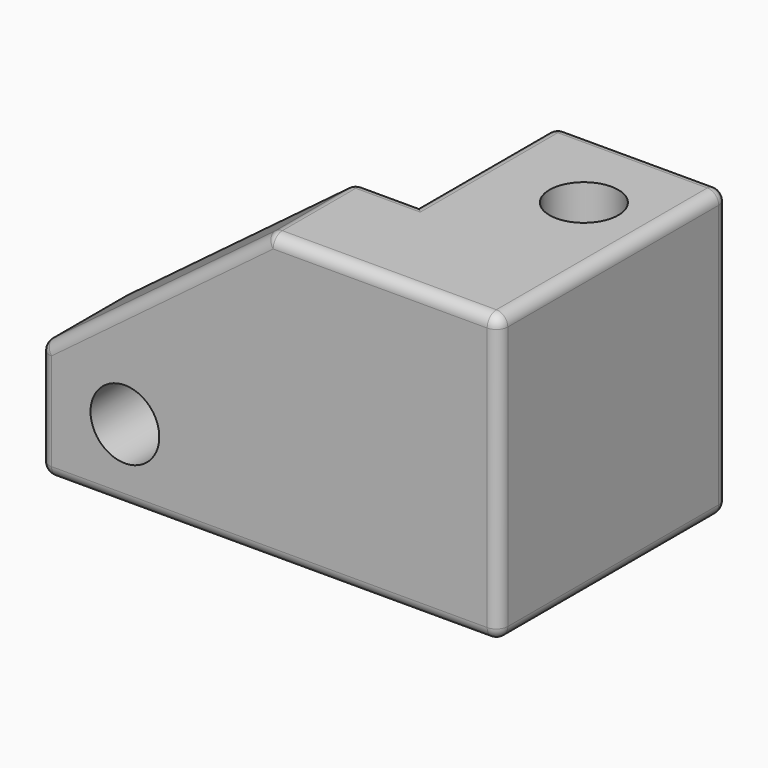
from build123d import *

# Parameters (mm, degrees)
F0_W          = 203.2
F0_H          = 127
F1_DEPTH      = 127
F3_DEPTH      = 76.2
F3_DEPTH_BACK = 76.2
F4_DEPTH      = 25.4
F5_SIZE2      = 101.6
F5_SIZE       = 76.2
F6_R          = 5.08
F7_R          = 15.24
F8_DEPTH      = 51.054
F9_R          = 15.24
F10_DEPTH     = 128.27


with BuildPart() as f1:
    # F0 (on Front) → F1 (new body)
    with BuildSketch(Plane.XZ):
        Rectangle(F0_W, F0_H)
    extrude(amount=F1_DEPTH)

    # F2 (on Front) → F3 (cut, two sides)
    with BuildSketch(Plane.XZ) as f3_sk:
        Polygon((25.2138410211, 63.1450035885), (-101.7861589789, 63.1450035885), (-101.7861589789, -63.8549964115), (-25.5861589789, -63.8549964115), (-25.5861589789, 12.3450035885), (25.2138410211, 12.3450035885), align=None)
    extrude(amount=-F3_DEPTH, mode=Mode.SUBTRACT)
    extrude(f3_sk.sketch, amount=F3_DEPTH_BACK, mode=Mode.SUBTRACT)

    # F4 (cut): a face of the model
    f4_faces = [f1.faces().sort_by_distance(p)[0] for p in [
        (-38.1930794895, -38.1, 63.1450035885),
    ]]
    extrude(f4_faces, amount=-F4_DEPTH, mode=Mode.SUBTRACT)

    # F5
    f5_edges = [f1.edges().sort_by_distance(p)[0] for p in [
        (-101.6, -101.6, 63.5),
    ]]
    f5_side = f1.faces().sort_by_distance((-101.6, -101.6, 0))[0]
    chamfer(f5_edges, length=F5_SIZE, length2=F5_SIZE2, reference=f5_side)

    # F6
    f6_edges = [f1.edges().sort_by_distance(p)[0] for p in [
        (25.213841, 0, 37.922502),
        (63.406921, 0, 63.5),
        (-0.186159, 0, 12.345004),
        (-25.586159, -38.1, 12.345004),
        (-101.6, -101.6, -12.7),
        (0, -101.6, 63.5),
        (101.6, 0, 0),
        (38.006921, 0, -63.5),
        (-25.586159, -38.1, -63.5),
        (-63.593079, -76.2, -63.5),
        (-101.6, -101.6, -63.5),
        (50.8, -127, 63.5),
        (-50.8, -127, 25.4),
        (101.6, -127, 0),
        (-101.6, -127, -38.1),
        (0, -127, -63.5),
        (-50.8, -76.2, 25.4),
        (101.6, -63.5, 63.5),
        (101.6, -63.5, -63.5),
        (12.606921, -76.2, 63.5),
        (25.213841, -38.1, 63.5),
    ]]
    fillet(f6_edges, radius=F6_R)

    # F7 (on face) → F8 (cut)
    with BuildSketch(Plane(origin=(0, -76.2, 0), x_dir=(-1, 0, 0), z_dir=(0, 1, 0))):
        with Locations((64.0217885375, -31.3331931829)):
            Circle(F7_R)
    extrude(amount=-F8_DEPTH, mode=Mode.SUBTRACT)

    # F9 (on face) → F10 (cut)
    with BuildSketch(Plane.XY.offset(63.5)):
        with Locations((69.9954107404, -40.2551107109)):
            Circle(F9_R)
    extrude(amount=-F10_DEPTH, mode=Mode.SUBTRACT)


solid = f1.part
